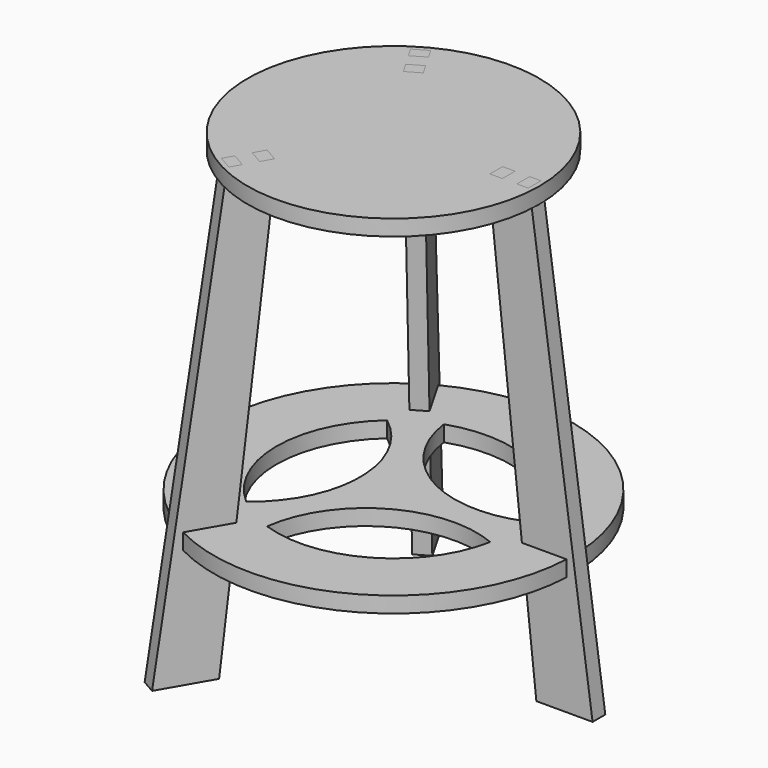
from build123d import *

# Parameters (mm, degrees)
F1_R      = 165.1
F2_DEPTH  = 17.9832
F4_R      = 203.2
F5_DEPTH  = 17.9832
F7_DEPTH  = 8.9916
F9_COUNT  = 3
F12_DEPTH = 17.9832


# Not quite as in the source:
# - a variable given as a bare number and used for a length is read in inches; the dataset says mm whatever the document's units were


with BuildPart() as f2:
    # F1 (on Top) → F2 (new body)
    with BuildSketch(Plane.XY):
        Circle(F1_R)
    extrude(amount=F2_DEPTH)


with BuildPart() as f5:
    # F4 (on offset) → F5 (new body)
    with BuildSketch(Plane.XY.offset(-355.6)):
        Circle(F4_R)
    extrude(amount=F5_DEPTH)


with BuildPart() as f7:
    # F6 (on Front) → F7 (new body, symmetric)
    with BuildSketch(Plane.XZ):
        Polygon((168.8860247109, -490.0168), (232.4975128982, -490.0168), (163.630142808, 0), (159.6704721451, 0), (159.6704721451, 17.9832), (146.8794196844, 17.9832), (146.8794196844, 0), (130.3748190403, 0), (130.3748190403, 17.9832), (116.3085358108, 17.9832), (116.3085358108, 0), (152.5339132969, -337.6168), (154.9490840925, -337.6168), (176.6884624437, -337.6168), (176.6884624437, -355.6), (154.4634624437, -355.6), align=None)
    extrude(amount=F7_DEPTH, both=True)


with BuildPart() as f9_1:
    # F9: instance of F7
    add(f7.part.rotate(Axis((0, 0, 58.8979013264), (0, 0, 1)), 1 * 360 / F9_COUNT))


with BuildPart() as f9_2:
    # F9: instance of F7
    add(f7.part.rotate(Axis((0, 0, 58.8979013264), (0, 0, 1)), 2 * 360 / F9_COUNT))


with BuildPart() as f2_1:
    add(f2.part)

    # F10: cut F7, F9_2, F9_1
    add(f7.part, mode=Mode.SUBTRACT)
    add(f9_2.part, mode=Mode.SUBTRACT)
    add(f9_1.part, mode=Mode.SUBTRACT)


with BuildPart() as f5_1:
    add(f5.part)

    # F10: cut F7, F9_2, F9_1
    add(f7.part, mode=Mode.SUBTRACT)
    add(f9_2.part, mode=Mode.SUBTRACT)
    add(f9_1.part, mode=Mode.SUBTRACT)

    # F11 (on face) → F12 (cut, through all)
    with BuildSketch(Plane.XY.offset(-337.6168)):
        with BuildLine():
            ThreePointArc((-42.9943574476, 125.0335251805), (18.7814760407, 32.5644928103), (129.7564533709, 25.4))
            ThreePointArc((129.7564533709, 25.4), (66.0577410848, 114.5350253598), (-42.9943574476, 125.0335251805))
        make_face()
        with BuildLine():
            ThreePointArc((-42.8811814293, -125.0723849242), (66.1613710423, -114.4751945759), (129.7793878548, -25.2825568213))
            ThreePointArc((129.7793878548, -25.2825568213), (18.8109400147, -32.547481777), (-42.8811814293, -125.0723849242))
        make_face()
        with BuildLine():
            ThreePointArc((-86.7850304073, -99.7509683592), (-37.5924160554, -0.0170110333), (-86.8752719416, 99.6723849242))
            ThreePointArc((-86.8752719416, 99.6723849242), (-132.2191121271, -0.0598307838), (-86.7850304073, -99.7509683592))
        make_face()
    extrude(amount=-F12_DEPTH, mode=Mode.SUBTRACT)


solid = Compound([f7.part, f9_1.part, f9_2.part, f2_1.part, f5_1.part])
